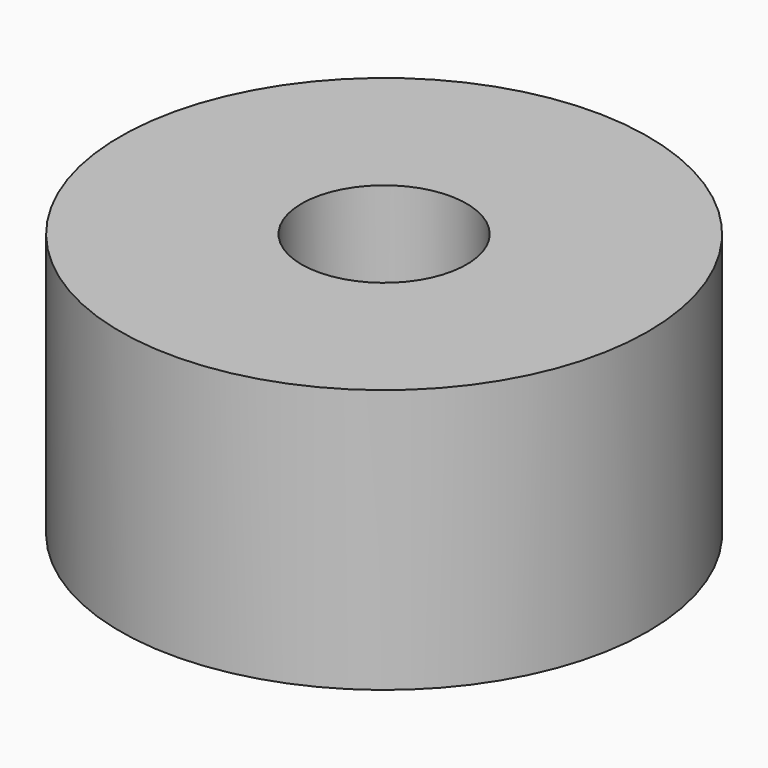
from build123d import *

# Parameters (mm, degrees)
F0_R     = 20
F1_DEPTH = 20
F2_D     = 12.5


with BuildPart() as f1:
    # F0 (on Top) → F1 (new body)
    with BuildSketch(Plane.XY):
        Circle(F0_R)
    extrude(amount=F1_DEPTH)

    # F2 (through all)
    with Locations(Plane(origin=(0, 0, 0), x_dir=(1, 0, 0), z_dir=(0, 0, -1))):
        with Locations((0, 0)):
            Hole(F2_D / 2)


solid = f1.part
